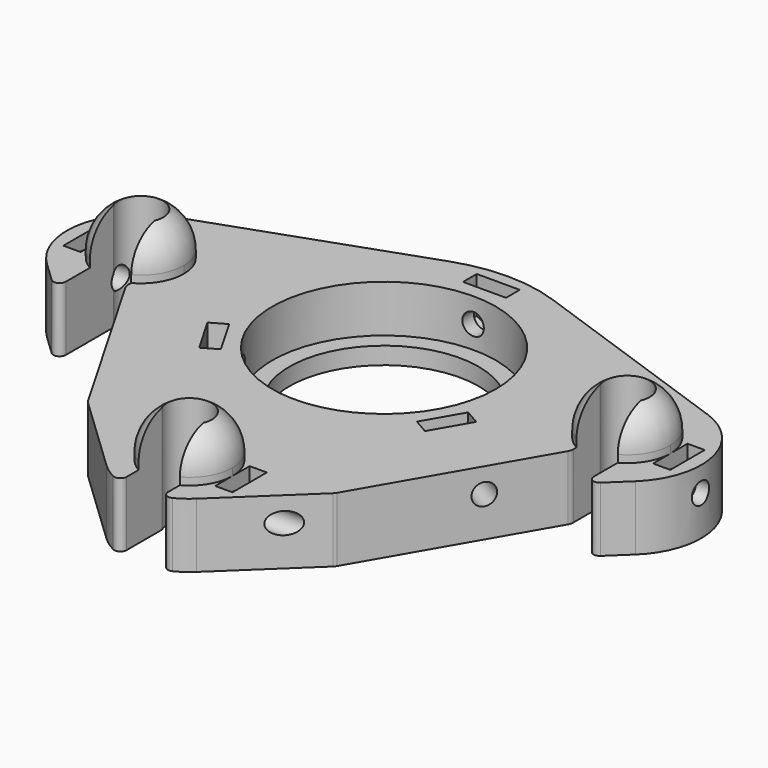
from build123d import *

# Parameters (mm, degrees)
F0_R         = 16.51
F1_DEPTH     = 9.525
F0_R_2       = 13.97
F2_DEPTH     = 2.54
F5_DEPTH     = 8.636
F6_T1_DEPTH  = 2.54
F6_T3_DEPTH  = 2.54
F6_T5_DEPTH  = 2.54
F6_T7_DEPTH  = 2.54
F6_T9_DEPTH  = 2.54
F6_T11_DEPTH = 2.54
F6_T13_DEPTH = 2.54
F6_T15_DEPTH = 2.54
F7_R         = 1.5875
F10_DEPTH    = 5.08
F8_R         = 1.5875
F11_DEPTH    = 20.32
F9_R         = 1.5875
F12_DEPTH    = 20.32
F13_DEPTH    = 6.35
F14_T2_ANGLE = 359.64
F14_T4_ANGLE = 359.64
F14_T6_ANGLE = 359.64
F17_R        = 1.5875
F18_DEPTH    = 6.35
F15_R        = 1.5875
F19_DEPTH    = 6.35
F16_R        = 1.5875
F20_DEPTH    = 7.62


# Not quite as in the source:
# - a fillet or chamfer that OpenCascade refuses, or shapes differently, is made with other operations: its cross-section is extruded or revolved along the edge and cut away or added


with BuildPart() as f1:
    # F0 (on Top) → F1 (new body)
    with BuildSketch(Plane.XY):
        with BuildLine():
            ThreePointArc((-3.048, -1.27), (0, 3.302), (3.048, -1.27))
            Line((3.048, -1.27), (3.048, -7.7856532174))
            ThreePointArc((3.048, -7.7856532174), (3.4850280464, -8.5661844882), (4.3788806587, -8.601541035))
            ThreePointArc((4.3788806587, -8.601541035), (5.5738439639, -7.8799344836), (6.6522190251, -6.9935031309))
            Line((6.6522190251, -6.9935031309), (18.1000873088, 3.8957072931))
            ThreePointArc((18.1000873088, 3.8957072931), (18.247113951, 4.0571486363), (18.3695596518, 4.2379446295))
            Line((18.3695596518, 4.2379446295), (32.6689376837, 29.0051938975))
            ThreePointArc((32.6689376837, 29.0051938975), (32.8211859276, 29.3727536727), (32.8731149683, 29.7671938975))
            Line((32.8731149683, 29.7671938975), (32.8731149683, 34.650934))
            ThreePointArc((32.8731149683, 34.650934), (35.9211149683, 39.222934), (38.9691149683, 34.650934))
            Line((38.9691149683, 34.650934), (38.9691149683, 25.8807274401))
            ThreePointArc((38.9691149683, 25.8807274401), (39.5237379199, 25.039336479), (40.5156301361, 25.2173679347))
            Line((40.5156301361, 25.2173679347), (43.4486259704, 28.0072330887))
            ThreePointArc((43.4486259704, 28.0072330887), (46.6013320921, 38.2063324748), (39.5509253491, 46.2221261931))
            Line((39.5509253491, 46.2221261931), (7.5972775411, 57.4815688228))
            ThreePointArc((7.5972775411, 57.4815688228), (0, 58.780934), (-7.5972775411, 57.4815688228))
            Line((-7.5972775411, 57.4815688228), (-39.5509253491, 46.2221261931))
            ThreePointArc((-39.5509253491, 46.2221261931), (-46.6013320921, 38.2063324748), (-43.4486259704, 28.0072330887))
            Line((-43.4486259704, 28.0072330887), (-40.5156301361, 25.2173679347))
            ThreePointArc((-40.5156301361, 25.2173679347), (-39.5237379199, 25.039336479), (-38.9691149683, 25.8807274401))
            Line((-38.9691149683, 25.8807274401), (-38.9691149683, 34.650934))
            ThreePointArc((-38.9691149683, 34.650934), (-35.9211149683, 39.222934), (-32.8731149683, 34.650934))
            Line((-32.8731149683, 34.650934), (-32.8731149683, 29.7671938975))
            ThreePointArc((-32.8731149683, 29.7671938975), (-32.8211859276, 29.3727536727), (-32.6689376837, 29.0051938975))
            Line((-32.6689376837, 29.0051938975), (-18.3695596518, 4.2379446295))
            ThreePointArc((-18.3695596518, 4.2379446295), (-18.247113951, 4.0571486363), (-18.1000873088, 3.8957072931))
            Line((-18.1000873088, 3.8957072931), (-6.6522190251, -6.9935031309))
            ThreePointArc((-6.6522190251, -6.9935031309), (-5.5738439639, -7.8799344836), (-4.3788806587, -8.601541035))
            ThreePointArc((-4.3788806587, -8.601541035), (-3.4850280464, -8.5661844882), (-3.048, -7.7856532174))
            Line((-3.048, -7.7856532174), (-3.048, -1.27))
        make_face()
        with Locations((0, 35.920934)):
            Circle(F0_R, mode=Mode.SUBTRACT)
    extrude(amount=F1_DEPTH)

    # F0 (on Top) → F2 (join)
    with BuildSketch(Plane.XY):
        with Locations((0, 35.920934)):
            Circle(F0_R)
        with Locations((0, 35.920934)):
            Circle(F0_R_2, mode=Mode.SUBTRACT)
    extrude(amount=F2_DEPTH)

    # F4 (on face) → F5 (cut)
    with BuildSketch(Plane.XY.offset(9.525)):
        Polygon((17.6453415423, 29.39956552), (14.4703415423, 23.900304206), (16.6700460679, 22.630304206), (19.8450460679, 28.12956552), align=None)
        Polygon((-3.175, 57.002932274), (-3.175, 54.462932274), (0, 54.462932274), (3.175, 54.462932274), (3.175, 57.002932274), align=None)
        Polygon((-14.4703415423, 23.900304206), (-17.6453415423, 29.39956552), (-19.8450460679, 28.12956552), (-16.6700460679, 22.630304206), align=None)
        Polygon((-42.2711149683, 32.745934), (-42.2711149683, 35.920934), (-42.2711149683, 39.095934), (-44.8111149683, 39.095934), (-44.8111149683, 32.745934), align=None)
        Polygon((42.2711149683, 39.095934), (42.2711149683, 35.920934), (42.2711149683, 32.745934), (44.8111149683, 32.745934), (44.8111149683, 39.095934), align=None)
        Polygon((6.35, 3.175), (6.35, 0), (6.35, -3.175), (8.89, -3.175), (8.89, 3.175), align=None)
    extrude(amount=-F5_DEPTH, mode=Mode.SUBTRACT)

    # F6: chamfer of 3.175 x 5.499261314 on 12 edges, made by hand

    # F6_s2 → F6_t1 (join)
    with BuildSketch(Plane(origin=(-0.5036208564, -0.290765637, 0), x_dir=(0, 0, 1), z_dir=(-0.8660254038, -0.5, 0))):
        Polygon((4.064, 34.2834413717), (0.889, 28.7841800576), (0.889, 34.2834413717), align=None)
    extrude(amount=F6_T1_DEPTH)

    # F6_s4 → F6_t3 (join)
    with BuildSketch(Plane(origin=(-2.703325382, -1.560765637, 0), x_dir=(0, 0, 1), z_dir=(0.8660254038, 0.5, 0))):
        Polygon((4.064, -27.9334413717), (0.889, -33.4327026857), (0.889, -27.9334413717), align=None)
    extrude(amount=F6_T3_DEPTH)

    # F6_s6 → F6_t5 (join)
    with BuildSketch(Plane.XZ.offset(-57.002932274)):
        Polygon((-3.175, 4.064), (2.324261314, 0.889), (-3.175, 0.889), align=None)
        Polygon((3.175, 4.064), (-2.324261314, 0.889), (3.175, 0.889), align=None)
    extrude(amount=F6_T5_DEPTH)

    # F6_s8 → F6_t7 (join)
    with BuildSketch(Plane(origin=(2.703325382, -1.560765637, 0), x_dir=(0, 0, 1), z_dir=(-0.8660254038, 0.5, 0))):
        Polygon((4.064, 34.2834413717), (0.889, 28.7841800576), (0.889, 34.2834413717), align=None)
    extrude(amount=F6_T7_DEPTH)

    # F6_s10 → F6_t9 (join)
    with BuildSketch(Plane(origin=(0.5036208564, -0.290765637, 0), x_dir=(0, 0, 1), z_dir=(0.8660254038, -0.5, 0))):
        Polygon((4.064, -27.9334413717), (0.889, -33.4327026857), (0.889, -27.9334413717), align=None)
    extrude(amount=F6_T9_DEPTH)

    # F6_s12 → F6_t11 (join)
    with BuildSketch(Plane.YZ.offset(-44.8111149683)):
        Polygon((39.095934, 4.064), (33.596672686, 0.889), (39.095934, 0.889), align=None)
        Polygon((32.745934, 4.064), (38.245195314, 0.889), (32.745934, 0.889), align=None)
    extrude(amount=F6_T11_DEPTH)

    # F6_s14 → F6_t13 (join)
    with BuildSketch(Plane.YZ.offset(6.35)):
        Polygon((3.175, 4.064), (-2.324261314, 0.889), (3.175, 0.889), align=None)
        Polygon((-3.175, 4.064), (2.324261314, 0.889), (-3.175, 0.889), align=None)
    extrude(amount=F6_T13_DEPTH)

    # F6_s16 → F6_t15 (join)
    with BuildSketch(Plane.YZ.offset(42.2711149683)):
        Polygon((39.095934, 4.064), (33.596672686, 0.889), (39.095934, 0.889), align=None)
        Polygon((32.745934, 4.064), (38.245195314, 0.889), (32.745934, 0.889), align=None)
    extrude(amount=F6_T15_DEPTH)

    # F7 (on face) → F10 (cut, symmetric)
    with BuildSketch(Plane.XZ.offset(-57.002932274)):
        with Locations((0, 5.8970871047)):
            Circle(F7_R)
    extrude(amount=F10_DEPTH, both=True, mode=Mode.SUBTRACT)

    # F8 (on face) → F11 (cut, symmetric)
    with BuildSketch(Plane(origin=(-2.703325382, -1.560765637, 0), x_dir=(-0.5, 0.8660254038, 0), z_dir=(0.8660254038, 0.5, 0))):
        with Locations((31.0334954411, 5.6098689985)):
            Circle(F8_R)
    extrude(amount=F11_DEPTH, both=True, mode=Mode.SUBTRACT)

    # F9 (on face) → F12 (cut, symmetric)
    with BuildSketch(Plane(origin=(2.703325382, -1.560765637, 0), x_dir=(-0.5, -0.8660254038, 0), z_dir=(-0.8660254038, 0.5, 0))):
        with Locations((-31.1158668548, 5.8928)):
            Circle(F9_R)
    extrude(amount=F12_DEPTH, both=True, mode=Mode.SUBTRACT)

    # F3 (on face) → F13 (join)
    with BuildSketch(Plane.XY.offset(9.525)):
        with BuildLine():
            ThreePointArc((-32.8731149683, 30.3502791013), (-30.4586384238, 32.6830566089), (-29.5711149683, 35.920934))
            ThreePointArc((-29.5711149683, 35.920934), (-39.1589923595, 41.3834105446), (-38.9691149683, 30.3502791013))
            Line((-38.9691149683, 30.3502791013), (-38.9691149683, 34.650934))
            ThreePointArc((-38.9691149683, 34.650934), (-35.9211149683, 39.222934), (-32.8731149683, 34.650934))
            Line((-32.8731149683, 34.650934), (-32.8731149683, 30.3502791013))
        make_face()
        with BuildLine():
            Line((38.9691149683, 34.650934), (38.9691149683, 30.3502791013))
            ThreePointArc((38.9691149683, 30.3502791013), (41.3835915129, 32.6830566089), (42.2711149683, 35.920934))
            ThreePointArc((42.2711149683, 35.920934), (32.6832375772, 41.3834105446), (32.8731149683, 30.3502791013))
            Line((32.8731149683, 30.3502791013), (32.8731149683, 34.650934))
            ThreePointArc((32.8731149683, 34.650934), (35.9211149683, 39.222934), (38.9691149683, 34.650934))
        make_face()
        with BuildLine():
            ThreePointArc((6.35, 0), (-3.2378773911, 5.4624765446), (-3.048, -5.5706548987))
            Line((-3.048, -5.5706548987), (-3.048, -1.27))
            ThreePointArc((-3.048, -1.27), (0, 3.302), (3.048, -1.27))
            Line((3.048, -1.27), (3.048, -5.5706548987))
            ThreePointArc((3.048, -5.5706548987), (5.4624765446, -3.2378773911), (6.35, 0))
        make_face()
    extrude(amount=F13_DEPTH)

    # F14: fillet of radius 6.096 on 3 edges, made by hand

    # F14_s1 → F14_t2 (revolve, cut)
    with BuildSketch(Plane(origin=(-35.8079122424, -0.1124942441, 0), x_dir=(0, 0, 1), z_dir=(-0.9999950652, -0.0031415875, 0))):
        with BuildLine():
            ThreePointArc((15.875, 32.7316060627), (13.6437091385, 30.5003152012), (10.5957091385, 29.6836060627))
            Line((10.5957091385, 29.6836060627), (15.875, 29.6836060627))
            Line((15.875, 29.6836060627), (15.875, 32.7316060627))
        make_face()
    revolve(axis=Axis((-35.9211149683, 35.920934, 15.875), (0, 0, 1)), revolution_arc=F14_T2_ANGLE, mode=Mode.SUBTRACT)

    # F14_s3 → F14_t4 (revolve, cut)
    with BuildSketch(Plane(origin=(36.0336086421, 0.1132032926, 0), x_dir=(0, 0, 1), z_dir=(-0.9999950652, -0.0031415875, 0))):
        with BuildLine():
            ThreePointArc((15.875, 32.5059074122), (13.6437091385, 30.2746165507), (10.5957091385, 29.4579074122))
            Line((10.5957091385, 29.4579074122), (15.875, 29.4579074122))
            Line((15.875, 29.4579074122), (15.875, 32.5059074122))
        make_face()
    revolve(axis=Axis((35.9211149683, 35.920934, 15.875), (0, 0, 1)), revolution_arc=F14_T4_ANGLE, mode=Mode.SUBTRACT)

    # F14_s5 → F14_t6 (revolve, cut)
    with BuildSketch(Plane(origin=(0, 0, 0), x_dir=(0, 0, 1), z_dir=(-0.9999950652, -0.0031415875, 0))):
        with BuildLine():
            ThreePointArc((15.875, -3.302), (13.6437091385, -5.5332908615), (10.5957091385, -6.35))
            Line((10.5957091385, -6.35), (15.875, -6.35))
            Line((15.875, -6.35), (15.875, -3.302))
        make_face()
    revolve(axis=Axis((0, 0, 15.875), (0, 0, 1)), revolution_arc=F14_T6_ANGLE, mode=Mode.SUBTRACT)

    # F17 (on face) → F18 (cut, symmetric)
    with BuildSketch(Plane(origin=(44.8111149683, 0, 0), x_dir=(0, -1, 0), z_dir=(-1, 0, 0))):
        with Locations((-35.9135085169, 5.8928)):
            Circle(F17_R)
    extrude(amount=F18_DEPTH, both=True, mode=Mode.SUBTRACT)

    # F15 (on face) → F19 (cut, symmetric)
    with BuildSketch(Plane.YZ.offset(-44.8111149683)):
        with Locations((35.9135085169, 5.8928)):
            Circle(F15_R)
    extrude(amount=F19_DEPTH, both=True, mode=Mode.SUBTRACT)

    # F16 (on face) → F20 (cut, symmetric)
    with BuildSketch(Plane(origin=(8.89, 0, 0), x_dir=(0, -1, 0), z_dir=(-1, 0, 0))):
        with Locations((0.0074254831, 5.8928)):
            Circle(F16_R)
    extrude(amount=F20_DEPTH, both=True, mode=Mode.SUBTRACT)


solid = f1.part
